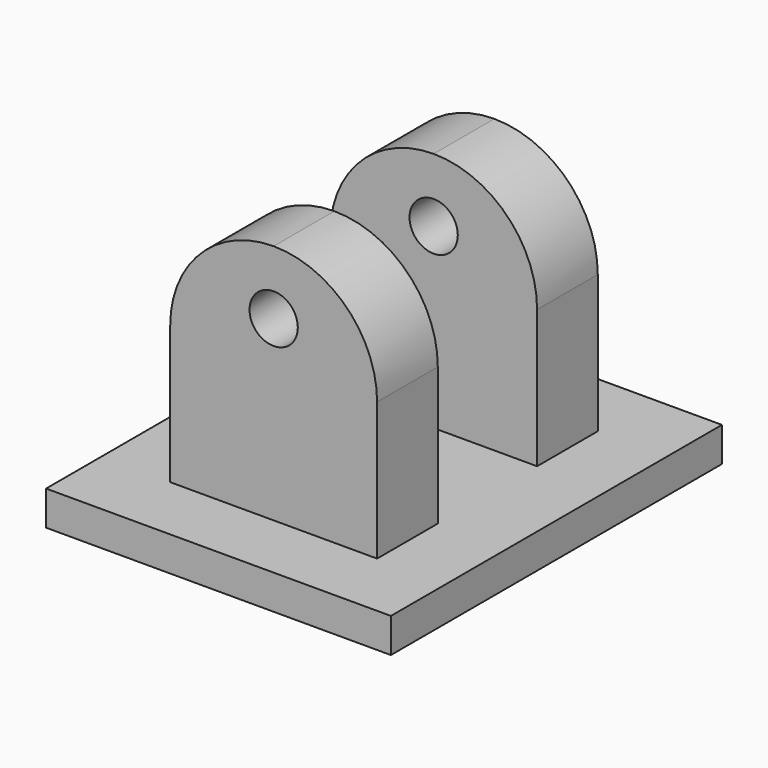
from build123d import *

# Parameters (mm, degrees)
F0_W     = 30
F0_H     = 11
F1_DEPTH = 40
F0_W_2   = 50
F0_H_2   = 60
F2_DEPTH = 5
F3_R     = 14.99999
F3_2_R   = 14.99999
F5_D     = 7
F5_2_D   = 7


# Not quite as in the source:
# - a fillet or chamfer is up to 0.001 mm smaller than in the source, because OpenCascade refuses the exact size


with BuildPart() as f1:
    # F0 (on Top) → F1 (new body)
    with BuildSketch(Plane.XY):
        with Locations((0, 14.5)):
            Rectangle(F0_W, F0_H)
    extrude(amount=F1_DEPTH)

    # F3#2 (radius 15 in the source; OpenCascade refuses exactly that, so slightly less here)
    f3_2_edges = [f1.edges().sort_by_distance(p)[0] for p in [
        (15, 14.5, 40),
        (-15, 14.5, 40),
    ]]
    fillet(f3_2_edges, radius=F3_2_R)

    # F5 (through all)
    with Locations(Plane(origin=(0, 20, 0), x_dir=(-1, 0, 0), z_dir=(0, 1, 0))):
        with Locations((0, 30.7527389377)):
            Hole(F5_D / 2)


with BuildPart() as f1b:
    # F0 (on Top) → F1, piece 2 (new body)
    with BuildSketch(Plane.XY):
        with Locations((0, -14.5)):
            Rectangle(F0_W, F0_H)
    extrude(amount=F1_DEPTH)

    # F3 (radius 15 in the source; OpenCascade refuses exactly that, so slightly less here)
    f3_edges = [f1b.edges().sort_by_distance(p)[0] for p in [
        (15, -14.5, 40),
        (-15, -14.5, 40),
    ]]
    fillet(f3_edges, radius=F3_R)

    # F5#2 (through all)
    with Locations(Plane(origin=(0, 20, 0), x_dir=(-1, 0, 0), z_dir=(0, 1, 0))):
        with Locations((0, 30.7527389377)):
            Hole(F5_2_D / 2)


with BuildPart() as f2:
    # F0 (on Top) → F2 (new body)
    with BuildSketch(Plane.XY):
        Rectangle(F0_W_2, F0_H_2)
        with Locations((0, -14.5)):
            Rectangle(F0_W, F0_H, mode=Mode.SUBTRACT)
        with Locations((0, 14.5)):
            Rectangle(F0_W, F0_H, mode=Mode.SUBTRACT)
    extrude(amount=F2_DEPTH)


solid = Compound([f1.part, f1b.part, f2.part])
